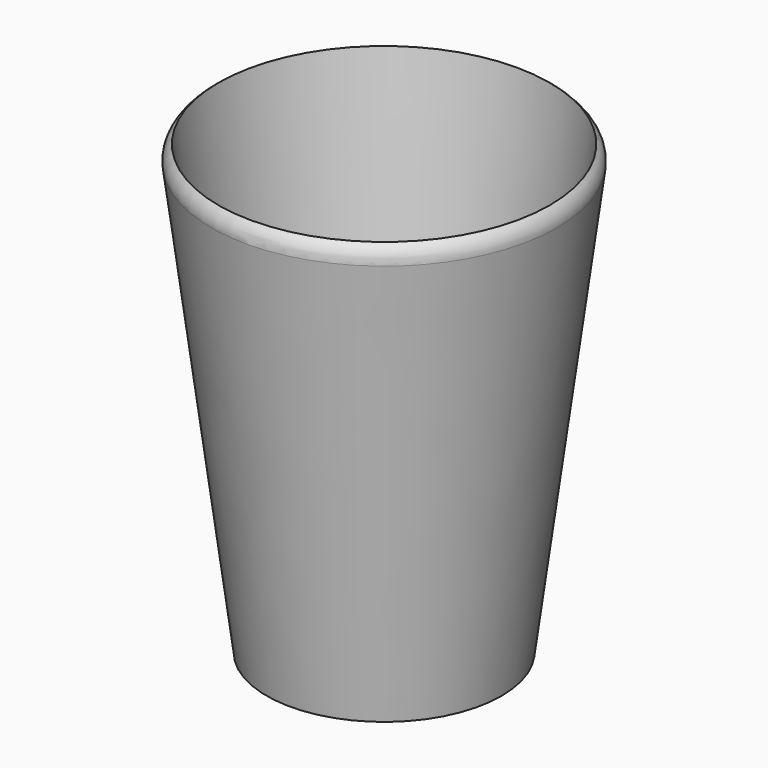
from build123d import *

# Parameters (mm, degrees)
F2_R = 46.99
F0_R = 31.496
F4_T = -2.54


# Not quite as in the source:
# - a fillet or chamfer that OpenCascade refuses, or shapes differently, is made with other operations: its cross-section is extruded or revolved along the edge and cut away or added


with BuildPart() as f3:
    # F2 (on offset) → F3 section 0
    with BuildSketch(Plane.XY.offset(119.99976)):
        Circle(F2_R)
    # F0 (on Top) → F3 section 1
    with BuildSketch(Plane.XY):
        Circle(F0_R)
    loft()

    # F4
    f4_openings = [f3.faces().sort_by_distance(p)[0] for p in [
        (0, 0, 119.99976),
    ]]
    offset(amount=F4_T, openings=f4_openings, kind=Kind.INTERSECTION)

    # F5: fillet of radius 5.08 on 1 edges, made by hand

    # F5_s1 → F5_t2 (revolve, cut)
    with BuildSketch(Plane.XZ):
        with BuildLine():
            ThreePointArc((46.3846421913, 115.3113133911), (46.0349113946, 117.9175544409), (44.4289151153, 119.99976))
            Line((44.4289151153, 119.99976), (46.99, 119.99976))
            Line((46.99, 119.99976), (46.3846421913, 115.3113133911))
        make_face()
    revolve(axis=Axis((0, 0, 119.99976), (0, 0, 1)), mode=Mode.SUBTRACT)


solid = f3.part
